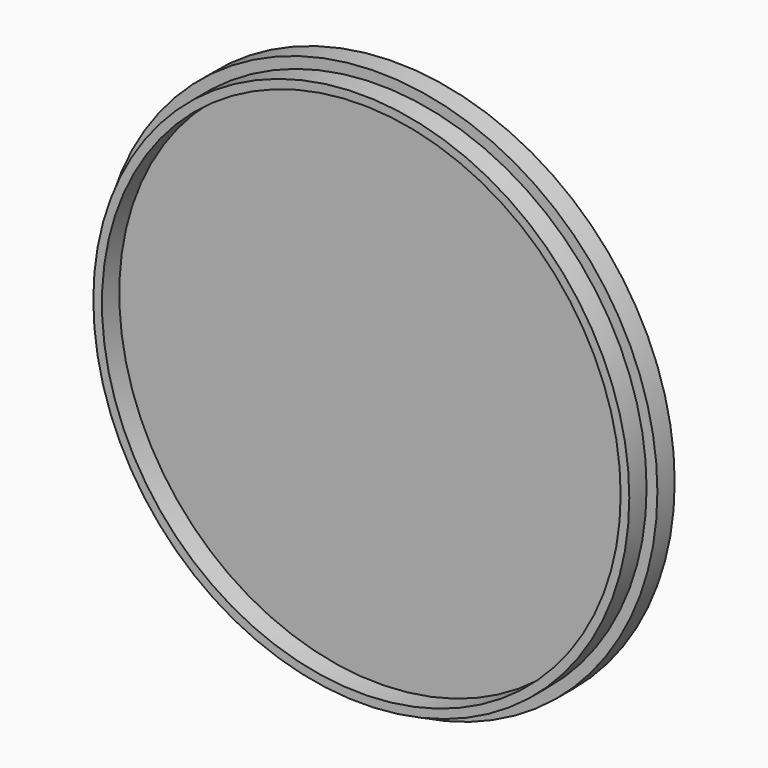
from build123d import *

# Parameters (mm, degrees)
F0_R     = 64.5
F0_R_2   = 62
F0_R_3   = 60
F1_DEPTH = 5
F2_DEPTH = 10


with BuildPart() as f1:
    # F0 (on Front) → F1 (new body)
    with BuildSketch(Plane.XZ):
        Circle(F0_R)
        Circle(F0_R_2, mode=Mode.SUBTRACT)
        Circle(F0_R_2)
        Circle(F0_R_3, mode=Mode.SUBTRACT)
        Circle(F0_R_3)
    extrude(amount=F1_DEPTH)

    # F0 (on Front) → F2 (join)
    with BuildSketch(Plane.XZ):
        Circle(F0_R_2)
        Circle(F0_R_3, mode=Mode.SUBTRACT)
    extrude(amount=F2_DEPTH)


solid = f1.part
